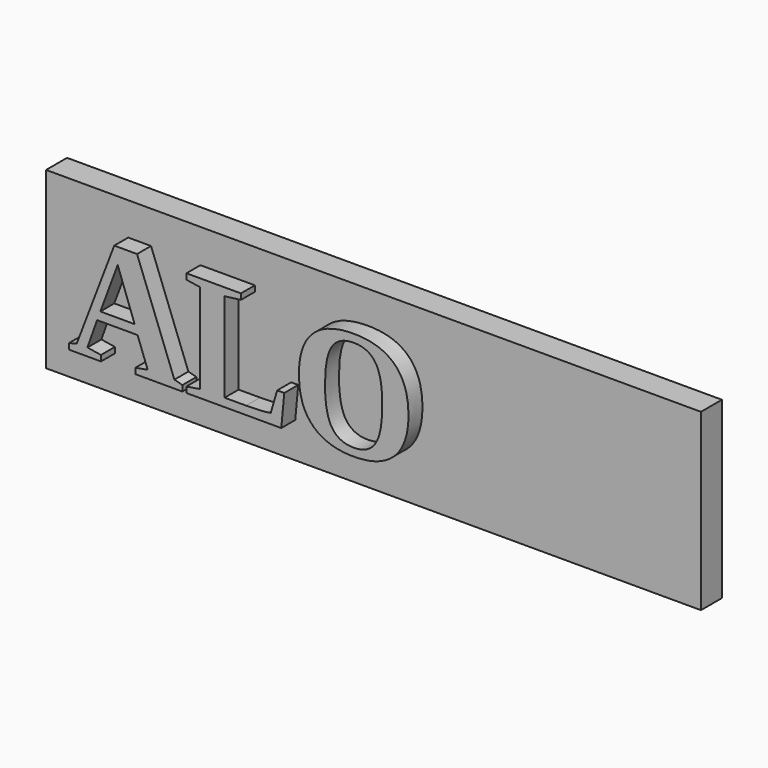
from build123d import *

# Parameters (mm, degrees)
F0_W         = 75
F0_H         = 20
F1_DEPTH     = 3
F2_TEXT_SIZE = 18.4443520589
F3_DEPTH     = 2


# Not quite as in the source:
# - Text() gives the source's letters only with a copy of the font that has no kerning and outlines rounded to 1/6400 em; it was checked with that copy


with BuildPart() as f1:
    # F0 (on Front) → F1 (new body)
    with BuildSketch(Plane.XZ):
        with Locations((37.4548381638, -10.1327993377)):
            Rectangle(F0_W, F0_H)
    extrude(amount=F1_DEPTH)

    # F2 (on face) → F3 (join)
    with BuildSketch(Plane.XZ.offset(3)):
        with Locations((3.9839800447, -16.0687193274)):
            Text('ALO', F2_TEXT_SIZE, font='Tinos', font_style=FontStyle.BOLD, text_align=(TextAlign.LEFT, TextAlign.BOTTOM))
    extrude(amount=F3_DEPTH)


solid = f1.part
